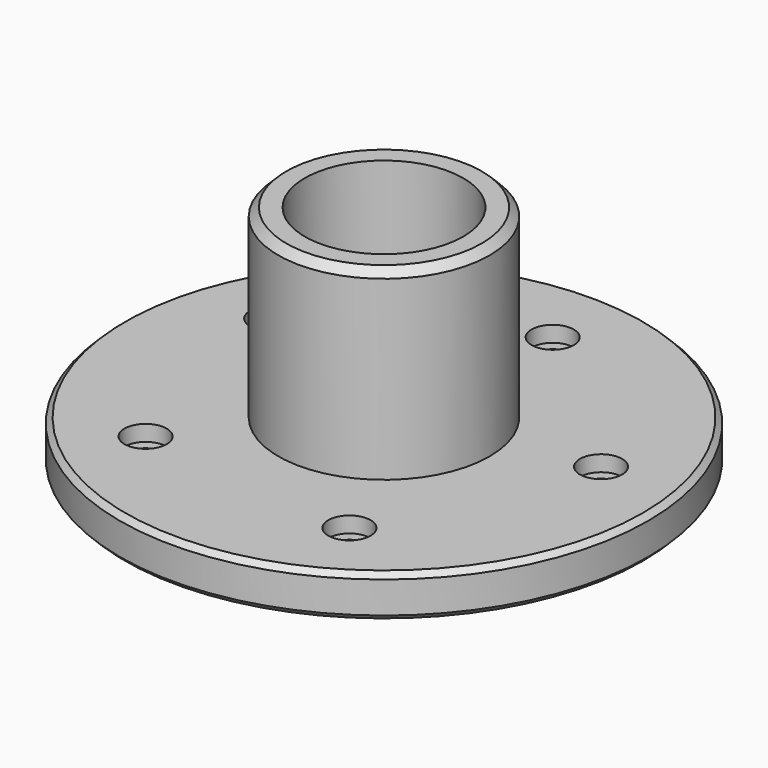
from build123d import *

# Parameters (mm, degrees)
F0_R            = 50
F1_DEPTH        = 8
F2_R            = 20
F3_DEPTH        = 35
F5_D            = 4
F5_DEPTH        = 12
F5_CBORE_D      = 8
F5_CBORE_DEPTH  = 3
F5_TIP          = 1.2017212381
F5_COPIES_COUNT = 5
F6_SIZE         = 1.5
F7_R            = 15
F8_DEPTH        = 43.001
F9_SIZE         = 1
F10_SIZE        = 1


# Not quite as in the source:
# - a pattern or mirror of a feature is missing from the dataset's text; its kind, count and spacing are read off the source's solid


with BuildPart() as f1:
    # F0 (on Top) → F1 (new body)
    with BuildSketch(Plane.XY):
        Circle(F0_R)
    extrude(amount=F1_DEPTH)

    # F2 (on face) → F3 (join)
    with BuildSketch(Plane.XY.offset(8)):
        Circle(F2_R)
    extrude(amount=F3_DEPTH)

    # F5
    with Locations(Plane.XY.offset(8)):
        with Locations((34.9212251604, 7.7109653503)):
            f5 = CounterBoreHole(F5_D / 2, F5_CBORE_D / 2, F5_CBORE_DEPTH, depth=F5_DEPTH)
            with Locations((0, 0, -(F5_DEPTH + F5_TIP / 2))):  # 118° drill point
                Cone(0, F5_D / 2, F5_TIP, mode=Mode.SUBTRACT)

    # F5_copies: F5 ×5 about axis
    f5_copies_axis = Axis((0, 0, 0), (0, 0, 1))
    for i in range(1, F5_COPIES_COUNT):
        add(f5.rotate(f5_copies_axis, i * 360 / F5_COPIES_COUNT), mode=Mode.SUBTRACT)

    # F6
    f6_edges = [f1.edges().sort_by_distance(p)[0] for p in [
        (-20, 0, 43),
    ]]
    chamfer(f6_edges, length=F6_SIZE)

    # F7 (on face) → F8 (cut, through all)
    with BuildSketch(Plane.XY.offset(43)):
        Circle(F7_R)
    extrude(amount=-F8_DEPTH, mode=Mode.SUBTRACT)

    # F9
    f9_edges = [f1.edges().sort_by_distance(p)[0] for p in [
        (-50, 0, 8),
        (-50, 0, 0),
    ]]
    chamfer(f9_edges, length=F9_SIZE)

    # F10
    f10_edges = [f1.edges().sort_by_distance(p)[0] for p in [
        (-15, 0, 0),
    ]]
    chamfer(f10_edges, length=F10_SIZE)


solid = f1.part
